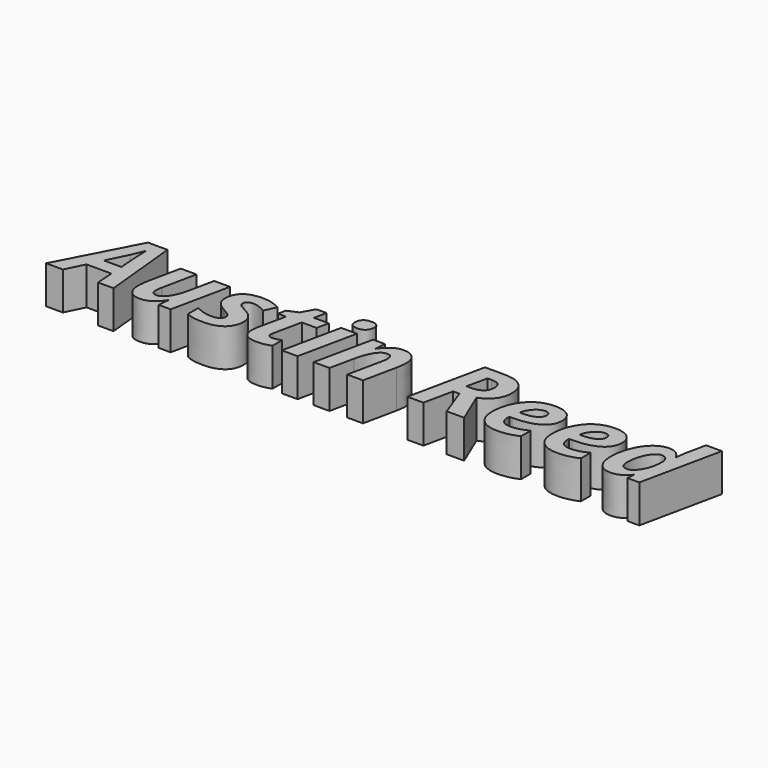
from build123d import *

# Parameters (mm, degrees)
F0_TEXT_SIZE = 72.0591956957
F1_DEPTH     = 25.4


# Not quite as in the source:
# - Text() gives the source's letters only with a copy of the font that has no kerning and outlines rounded to 1/6400 em; it was checked with that copy


with BuildPart() as f1:
    # F0 (on Top) → F1 (new body)
    with BuildSketch(Plane.XY):
        with Locations((-83.0704942346, -18.2172134519)):
            Text('Austin Reed', F0_TEXT_SIZE, font='Open Sans', font_style=FontStyle.BOLDITALIC, text_align=(TextAlign.LEFT, TextAlign.BOTTOM))
    extrude(amount=F1_DEPTH)


solid = f1.part
